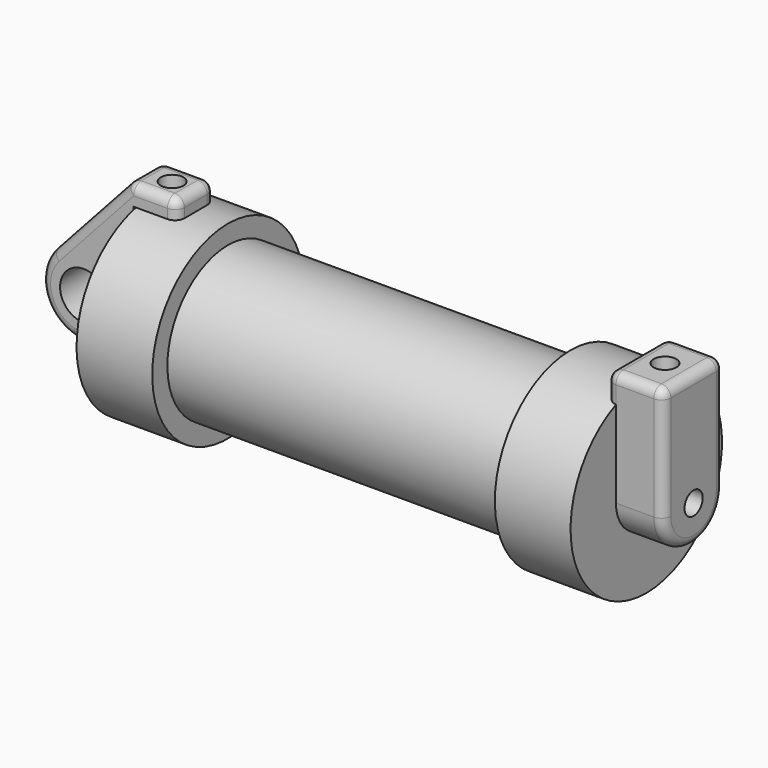
from build123d import *
from build123d import SkipClean  # not in build123d's __all__

# Parameters (mm, degrees)
F0_W      = 5.842
F0_H      = 12.7
F0_R      = 3.175
F2_DEPTH  = 3.175
F4_DEPTH  = 60.452
F5_R      = 1.524
F6_DEPTH  = 1.27
F7_DEPTH  = 6.35
F10_DEPTH = 17.78
F11_R     = 1.524
F12_DEPTH = 10.414
F13_R     = 1.27
F14_R     = 1.27


# Not quite as in the source:
# - after a boolean that leaves OpenCascade's solid faulty, fix() repairs it


with BuildPart() as f1:
    # F0 (on Front) → F1 (revolve)
    with BuildSketch(Plane.XZ):
        Polygon((5.842, 12.7), (5.842, 0), (66.294, 0), (66.294, 12.7), (56.134, 12.7), (56.134, 10.16), (10.16, 10.16), (10.16, 12.7), align=None)
        with Locations((2.921, 6.35)):
            Rectangle(F0_W, F0_H)
    revolve(axis=Axis((33.147, 0, 0), (-1, 0, 0)))

    # F3 (on face) → F4 (cut)
    with BuildSketch(Plane.YZ.offset(66.294)):
        with BuildLine():
            Line((-1.524, 0), (1.524, 0))
            ThreePointArc((1.524, 0), (0, 1.524), (-1.524, 0))
        make_face()
        with BuildLine():
            ThreePointArc((-1.524, 0), (0, -1.524), (1.524, 0))
            Line((1.524, 0), (-1.524, 0))
        make_face()
    extrude(amount=-F4_DEPTH, mode=Mode.SUBTRACT)

    # F5 (on face) → F6 (join)
    with BuildSketch(Plane.YZ.offset(66.294)):
        with BuildLine():
            ThreePointArc((-5.08, 0), (0, 5.08), (5.08, 0))
            Line((5.08, 0), (5.08, 11.6397422652))
            ThreePointArc((5.08, 11.6397422652), (0, 12.7), (-5.08, 11.6397422652))
            Line((-5.08, 11.6397422652), (-5.08, 0))
        make_face()
        with BuildLine():
            ThreePointArc((-5.08, 11.6397422652), (0, 12.7), (5.08, 11.6397422652))
            Line((5.08, 11.6397422652), (5.08, 15.24))
            Line((5.08, 15.24), (-5.08, 15.24))
            Line((-5.08, 15.24), (-5.08, 11.6397422652))
        make_face()
        with BuildLine():
            ThreePointArc((-5.08, 0), (0, -5.08), (5.08, 0))
            ThreePointArc((5.08, 0), (0, 5.08), (-5.08, 0))
        make_face()
        Circle(F5_R, mode=Mode.SUBTRACT)
    extrude(amount=-F6_DEPTH)

    # F5 (on face) → F7 (join)
    with BuildSketch(Plane.YZ.offset(66.294)):
        with BuildLine():
            ThreePointArc((-5.08, 0), (0, 5.08), (5.08, 0))
            Line((5.08, 0), (5.08, 11.6397422652))
            ThreePointArc((5.08, 11.6397422652), (0, 12.7), (-5.08, 11.6397422652))
            Line((-5.08, 11.6397422652), (-5.08, 0))
        make_face()
        with BuildLine():
            ThreePointArc((-5.08, 11.6397422652), (0, 12.7), (5.08, 11.6397422652))
            Line((5.08, 11.6397422652), (5.08, 15.24))
            Line((5.08, 15.24), (-5.08, 15.24))
            Line((-5.08, 15.24), (-5.08, 11.6397422652))
        make_face()
        with BuildLine():
            ThreePointArc((-5.08, 0), (0, -5.08), (5.08, 0))
            ThreePointArc((5.08, 0), (0, 5.08), (-5.08, 0))
        make_face()
        Circle(F5_R, mode=Mode.SUBTRACT)
    with SkipClean():  # cleaning this boolean's faces spoils the solid; the shape is the same uncleaned
        extrude(amount=F7_DEPTH)

    # F11 (on face) → F12 (cut)
    with BuildSketch(Plane.XY.offset(15.24)):
        with Locations((68.7653996064, 0.0510123878)):
            Circle(F11_R)
    extrude(amount=-F12_DEPTH, mode=Mode.SUBTRACT)

    add(f1.part.fix(), mode=Mode.REPLACE)

    # F13
    f13_edges = [f1.edges().sort_by_distance(p)[0] for p in [
        (72.644, -5.08, 7.62),
        (68.834, -5.08, 15.24),
        (72.644, 0, 15.24),
        (65.024, 0, 15.24),
        (68.834, 5.08, 15.24),
        (65.024, -5.08, 13.439871),
        (65.024, 5.08, 13.439871),
    ]]
    fillet(f13_edges, radius=F13_R)


with BuildPart() as f2:
    # F0 (on Front) → F2 (new body, symmetric)
    with BuildSketch(Plane.XZ):
        with BuildLine():
            Line((-0.9398, 0), (0, 0))
            Line((0, 0), (0, 12.7))
            Line((0, 12.7), (5.842, 12.7))
            Line((5.842, 12.7), (5.842, 15.24))
            Line((5.842, 15.24), (-0.508, 15.24))
            Line((-0.508, 15.24), (-10.8806298187, 3.8475430269))
            ThreePointArc((-10.8806298187, 3.8475430269), (-4.5919612295, 5.3297205562), (-0.9398, 0))
        make_face()
        with BuildLine():
            ThreePointArc((-8.1826630726, -5.5069827884), (-3.1957909266, -4.5493385486), (-0.9398, 0))
            ThreePointArc((-0.9398, 0), (-4.5919612295, 5.3297205562), (-10.8806298187, 3.8475430269))
            ThreePointArc((-10.8806298187, 3.8475430269), (-12.1459778134, -1.5837270034), (-8.1826630726, -5.5069827884))
        make_face()
        with Locations((-6.6548, 0)):
            Circle(F0_R, mode=Mode.SUBTRACT)
        with BuildLine():
            Line((5.842, 0), (0, 0))
            Line((0, 0), (-0.9398, 0))
            ThreePointArc((-0.9398, 0), (-3.1957909266, -4.5493385486), (-8.1826630726, -5.5069827884))
            Line((-8.1826630726, -5.5069827884), (5.842, -9.398))
            Line((5.842, -9.398), (5.842, 0))
        make_face()
    extrude(amount=F2_DEPTH, both=True)

    # F9 (on face) → F10 (cut)
    with BuildSketch(Plane.XY.offset(15.24)):
        with BuildLine():
            ThreePointArc((4.191, 0), (2.667, 1.524), (1.143, 0))
            ThreePointArc((1.143, 0), (2.667, -1.524), (4.191, 0))
        make_face()
    extrude(amount=-F10_DEPTH, mode=Mode.SUBTRACT)

    # F14
    f14_edges = [f2.edges().sort_by_distance(p)[0] for p in [
        (-5.694315, -3.175, 9.543772),
        (-5.694315, 3.175, 9.543772),
        (-0.508, 0, 15.24),
        (2.667, 3.175, 15.24),
        (5.842, 3.175, 13.97),
        (5.842, 0, 15.24),
        (2.667, -3.175, 15.24),
        (5.842, -3.175, 13.97),
        (-12.145978, 3.175, -1.583727),
        (-1.170332, 3.175, -7.452491),
        (-12.145978, -3.175, -1.583727),
        (-1.170332, -3.175, -7.452491),
    ]]
    fillet(f14_edges, radius=F14_R)


solid = Compound([f1.part, f2.part])
